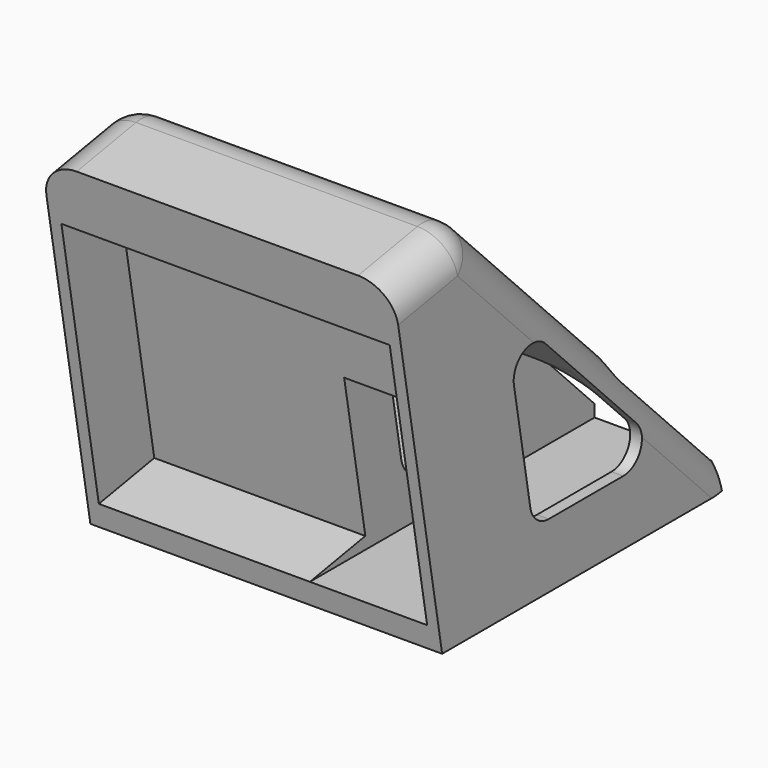
from build123d import *

# Parameters (mm, degrees)
F0_W          = 30
F0_H          = 30
F4_DEPTH      = 3
F3_W          = 30
F3_H          = 30
F5_DEPTH      = 8
F6_DEPTH      = 25
F8_DEPTH      = 6.0000000522
F10_DEPTH     = 30
F7_W          = 10
F7_H          = 11.7721162952
F7_H_2        = 1.030384494
F11_DEPTH     = 35.21044533
F12_T4_DEPTH  = 18.4976166065
F12_T10_DEPTH = 18.4976166065
F12_T15_DEPTH = 17.5385665297
F12_T20_DEPTH = 17.5385665297
F12_T26_DEPTH = 17.5385665297
F12_T31_DEPTH = 17.5385665297
F12_T37_DEPTH = 18.4976166065
F12_T43_DEPTH = 18.4976166065
F12_T45_DEPTH = 13.9174578279
F12_T47_DEPTH = 24
F12_T49_DEPTH = 44.997612514
F12_T54_DEPTH = 3
F12_T60_DEPTH = 3
F3_W_2        = 10
F3_H_2        = 13
F13_DEPTH     = 5.1313021672
F14_DEPTH     = 10.5


# Not quite as in the source:
# - a fillet or chamfer that OpenCascade refuses, or shapes differently, is made with other operations: its cross-section is extruded or revolved along the edge and cut away or added


with BuildPart() as f4:
    # F0 (on Top) → F4 (new body)
    with BuildSketch(Plane.XY):
        with Locations((0, 15)):
            Rectangle(F0_W, F0_H)
    extrude(amount=F4_DEPTH)

    # F3 (on 3pt) → F5 (join)
    with BuildSketch(Plane(origin=(0, 0, 0), x_dir=(-1, 0, 0), z_dir=(0, 0.984807753, 0.1736481777))):
        with Locations((0, 15)):
            Rectangle(F3_W, F3_H)
        Polygon((-14, 2), (-14, 15), (-14, 25), (14, 25), (14, 2), (-4, 2), align=None, mode=Mode.SUBTRACT)
        Polygon((-14, 25), (-14, 15), (-4, 15), (-4, 2), (14, 2), (14, 25), align=None)
    extrude(amount=F5_DEPTH)

    # F0 (on Top) → F6 (cut)
    with BuildSketch(Plane.XY):
        with Locations((0, 15)):
            Rectangle(F0_W, F0_H)
    extrude(amount=-F6_DEPTH, mode=Mode.SUBTRACT)

    # F3 (on 3pt) → F8 (cut)
    with BuildSketch(Plane(origin=(0, 0, 0), x_dir=(-1, 0, 0), z_dir=(0, 0.984807753, 0.1736481777))):
        Polygon((-14, 25), (-14, 15), (-4, 15), (-4, 2), (14, 2), (14, 25), align=None)
    extrude(amount=F8_DEPTH, mode=Mode.SUBTRACT)

    # F9 (on face) → F10 (join, through all)
    with BuildSketch(Plane.YZ.offset(15)):
        Polygon((30, 3), (2.6690166941, 30.9334180117), (7.594431953, 3), align=None)
        with BuildLine():
            ThreePointArc((11.3703802933, 5.5), (10.0848050739, 5.9679111138), (9.4007647872, 7.1527036447))
            Line((9.4007647872, 7.1527036447), (7.6573020205, 17.0403723366))
            ThreePointArc((7.6573020205, 17.0403723366), (8.7131028501, 19.1666972856), (11.0564624317, 18.7863828744))
            Line((11.0564624317, 18.7863828744), (20.7308856563, 8.8987141825))
            ThreePointArc((20.7308856563, 8.8987141825), (21.1449009434, 6.7245737833), (19.3013407511, 5.5))
            Line((19.3013407511, 5.5), (11.3703802933, 5.5))
        make_face(mode=Mode.SUBTRACT)
    extrude(amount=-F10_DEPTH)

    # F7 (on face) → F11 (cut, through all)
    with BuildSketch(Plane(origin=(0, 30, 0), x_dir=(-1, 0, 0), z_dir=(0, 1, 0))):
        with Locations((-9, 8.8860581476)):
            Rectangle(F7_W, F7_H)
        with Locations((-9, 2.484807753)):
            Rectangle(F7_W, F7_H_2)
    extrude(amount=-F11_DEPTH, mode=Mode.SUBTRACT)

    # F12: fillet of radius 3 on 9 edges, made by hand


with BuildPart() as f12_tool2:
    # F12_s3 → F12_t4 (new body)
    with BuildSketch(Plane.XZ.offset(-25.9817706947)):
        with BuildLine():
            ThreePointArc((7, 14.7721162952), (4.8786796564, 13.8934366387), (4, 11.7721162952))
            Line((4, 11.7721162952), (4, 14.7721162952))
            Line((4, 14.7721162952), (7, 14.7721162952))
        make_face()
    extrude(amount=F12_T4_DEPTH)

    split(bisect_by=Plane(origin=(0, 16.8266333185, 16.4637365227), x_dir=(1, 0, 0), z_dir=(0, -0.7147724526, -0.6993570912)), keep=Keep.TOP)

    split(bisect_by=Plane(origin=(0, 15.0397021871, 14.7153437946), x_dir=(1, 0, 0), z_dir=(0, 0.7147724526, 0.6993570912)), keep=Keep.TOP)


with BuildPart() as f4_1:
    add(f4.part)

    # F12_t1: union F12_tool2
    add(f12_tool2.part)


with BuildPart() as f12_tool8:
    # F12_s9 → F12_t10 (new body)
    with BuildSketch(Plane.XZ.offset(-25.9817706947)):
        with BuildLine():
            ThreePointArc((7, 14.7721162952), (4.8786796564, 13.8934366387), (4, 11.7721162952))
            Line((4, 11.7721162952), (4, 14.7721162952))
            Line((4, 14.7721162952), (7, 14.7721162952))
        make_face()
    extrude(amount=F12_T10_DEPTH)

    split(bisect_by=Plane(origin=(0, 10.3404814066, 1.8233058655), x_dir=(1, 0, 0), z_dir=(0, -0.984807753, -0.1736481777)), keep=Keep.TOP)


with BuildPart() as f4_2:
    add(f4_1.part)

    # F12_t7: union F12_tool8
    add(f12_tool8.part)


with BuildPart() as f12_tool13:
    # F12_s14 → F12_t15 (new body)
    with BuildSketch(Plane.XZ.offset(-15.5572567598)):
        with BuildLine():
            ThreePointArc((7, 14.7721162952), (4.8786796564, 13.8934366387), (4, 11.7721162952))
            Line((4, 11.7721162952), (4, 14.7721162952))
            Line((4, 14.7721162952), (7, 14.7721162952))
        make_face()
    extrude(amount=F12_T15_DEPTH)

    split(bisect_by=Plane(origin=(0, 15.0397021871, 14.7153437946), x_dir=(1, 0, 0), z_dir=(0, 0.7147724526, 0.6993570912)), keep=Keep.TOP)


with BuildPart() as f4_3:
    add(f4_2.part)

    # F12_t12: union F12_tool13
    add(f12_tool13.part)


with BuildPart() as f12_tool18:
    # F12_s19 → F12_t20 (new body)
    with BuildSketch(Plane.XZ.offset(-15.5572567598)):
        with BuildLine():
            ThreePointArc((7, 14.7721162952), (4.8786796564, 13.8934366387), (4, 11.7721162952))
            Line((4, 11.7721162952), (4, 14.7721162952))
            Line((4, 14.7721162952), (7, 14.7721162952))
        make_face()
    extrude(amount=F12_T20_DEPTH)

    split(bisect_by=Plane(origin=(0, 10.3404814066, 1.8233058655), x_dir=(1, 0, 0), z_dir=(0, -0.984807753, -0.1736481777)), keep=Keep.TOP)

    split(bisect_by=Plane(origin=(0, 7.8784620241, 1.3891854213), x_dir=(1, 0, 0), z_dir=(0, 0.984807753, 0.1736481777)), keep=Keep.TOP)


with BuildPart() as f4_4:
    add(f4_3.part)

    # F12_t17: union F12_tool18
    add(f12_tool18.part)


with BuildPart() as f12_tool24:
    # F12_s25 → F12_t26 (new body)
    with BuildSketch(Plane.XZ.offset(-15.5572567598)):
        with BuildLine():
            ThreePointArc((14, 11.7721162952), (13.1213203436, 13.8934366387), (11, 14.7721162952))
            Line((11, 14.7721162952), (14, 14.7721162952))
            Line((14, 14.7721162952), (14, 11.7721162952))
        make_face()
    extrude(amount=F12_T26_DEPTH)

    split(bisect_by=Plane(origin=(0, 15.0397021871, 14.7153437946), x_dir=(1, 0, 0), z_dir=(0, 0.7147724526, 0.6993570912)), keep=Keep.TOP)


with BuildPart() as f4_5:
    add(f4_4.part)

    # F12_t23: union F12_tool24
    add(f12_tool24.part)


with BuildPart() as f12_tool29:
    # F12_s30 → F12_t31 (new body)
    with BuildSketch(Plane.XZ.offset(-15.5572567598)):
        with BuildLine():
            ThreePointArc((14, 11.7721162952), (13.1213203436, 13.8934366387), (11, 14.7721162952))
            Line((11, 14.7721162952), (14, 14.7721162952))
            Line((14, 14.7721162952), (14, 11.7721162952))
        make_face()
    extrude(amount=F12_T31_DEPTH)

    split(bisect_by=Plane(origin=(0, 10.3404814066, 1.8233058655), x_dir=(1, 0, 0), z_dir=(0, -0.984807753, -0.1736481777)), keep=Keep.TOP)

    split(bisect_by=Plane(origin=(0, 7.8784620241, 1.3891854213), x_dir=(1, 0, 0), z_dir=(0, 0.984807753, 0.1736481777)), keep=Keep.TOP)


with BuildPart() as f4_6:
    add(f4_5.part)

    # F12_t28: union F12_tool29
    add(f12_tool29.part)


with BuildPart() as f12_tool35:
    # F12_s36 → F12_t37 (new body)
    with BuildSketch(Plane.XZ.offset(-25.9817706947)):
        with BuildLine():
            ThreePointArc((14, 11.7721162952), (13.1213203436, 13.8934366387), (11, 14.7721162952))
            Line((11, 14.7721162952), (14, 14.7721162952))
            Line((14, 14.7721162952), (14, 11.7721162952))
        make_face()
    extrude(amount=F12_T37_DEPTH)

    split(bisect_by=Plane(origin=(0, 16.8266333185, 16.4637365227), x_dir=(1, 0, 0), z_dir=(0, -0.7147724526, -0.6993570912)), keep=Keep.TOP)

    split(bisect_by=Plane(origin=(0, 15.0397021871, 14.7153437946), x_dir=(1, 0, 0), z_dir=(0, 0.7147724526, 0.6993570912)), keep=Keep.TOP)


with BuildPart() as f4_7:
    add(f4_6.part)

    # F12_t34: union F12_tool35
    add(f12_tool35.part)


with BuildPart() as f12_tool41:
    # F12_s42 → F12_t43 (new body)
    with BuildSketch(Plane.XZ.offset(-25.9817706947)):
        with BuildLine():
            ThreePointArc((14, 11.7721162952), (13.1213203436, 13.8934366387), (11, 14.7721162952))
            Line((11, 14.7721162952), (14, 14.7721162952))
            Line((14, 14.7721162952), (14, 11.7721162952))
        make_face()
    extrude(amount=F12_T43_DEPTH)

    split(bisect_by=Plane(origin=(0, 10.3404814066, 1.8233058655), x_dir=(1, 0, 0), z_dir=(0, -0.984807753, -0.1736481777)), keep=Keep.TOP)


with BuildPart() as f4_8:
    add(f4_7.part)

    # F12_t40: union F12_tool41
    add(f12_tool41.part)

    # F12_s46 → F12_t45 (cut)
    with BuildSketch(Plane(origin=(0, -7.3860581476, -1.3023613325), x_dir=(1, 0, 0), z_dir=(0, 0.984807753, 0.1736481777))):
        with BuildLine():
            ThreePointArc((-15, -27), (-14.1213203436, -29.1213203436), (-12, -30))
            Line((-12, -30), (-15, -30))
            Line((-15, -30), (-15, -27))
        make_face()
        with BuildLine():
            ThreePointArc((15, -27), (14.1213203436, -29.1213203436), (12, -30))
            Line((12, -30), (15, -30))
            Line((15, -30), (15, -27))
        make_face()
    extrude(amount=F12_T45_DEPTH, mode=Mode.SUBTRACT)

    # F12_s48 → F12_t47 (cut)
    with BuildSketch(Plane.YZ.offset(-12)):
        with BuildLine():
            ThreePointArc((1.1105168936, 30.6586124474), (2.5491593686, 30.5603807939), (3.7757787843, 29.8022604621))
            Line((3.7757787843, 29.8022604621), (2.6690166941, 30.9334180117))
            Line((2.6690166941, 30.9334180117), (1.1105168936, 30.6586124474))
        make_face()
    extrude(amount=F12_T47_DEPTH, mode=Mode.SUBTRACT)

    # F12_s50 → F12_t49 (cut)
    with BuildSketch(Plane(origin=(0, 18.4185448657, -18.8245299169), x_dir=(1, 0, 0), z_dir=(0, -0.6993570912, 0.7147724526))):
        with BuildLine():
            ThreePointArc((-15, 20.5412448507), (-14.1213203436, 22.6625651943), (-12, 23.5412448507))
            Line((-12, 23.5412448507), (-15, 23.5412448507))
            Line((-15, 23.5412448507), (-15, 20.5412448507))
        make_face()
        with BuildLine():
            ThreePointArc((15, 20.5412448507), (14.1213203436, 22.6625651943), (12, 23.5412448507))
            Line((12, 23.5412448507), (15, 23.5412448507))
            Line((15, 23.5412448507), (15, 20.5412448507))
        make_face()
    extrude(amount=F12_T49_DEPTH, mode=Mode.SUBTRACT)


with BuildPart() as f12_tool52:
    # F12_s53 → F12_t54 (new body)
    with BuildSketch(Plane.YZ.offset(-12)):
        Polygon((1.6314614266, 27.7041891884), (1.1105168936, 30.6586124474), (2.6690166941, 30.9334180117), (3.7757787843, 29.8022604621), align=None)
    extrude(amount=-F12_T54_DEPTH)

    # F12_s55 → F12_t56 (revolve, cut)
    with BuildSketch(Plane(origin=(-12, 1.6314614266, 27.7041891884), x_dir=(0, -0.305899314, -0.9520638685), z_dir=(0, 0.9520638685, -0.305899314))):
        with BuildLine():
            ThreePointArc((0, -3), (3, 0), (0, 3))
            Line((0, 3), (0, -3))
        make_face()
    revolve(axis=Axis((-12, 1.6314614266, 27.7041891884), (-1, 0, 0)), mode=Mode.SUBTRACT)


with BuildPart() as f4_9:
    add(f4_8.part)

    # F12_t51: cut F12_tool52
    add(f12_tool52.part, mode=Mode.SUBTRACT)


with BuildPart() as f12_tool58:
    # F12_s59 → F12_t60 (new body)
    with BuildSketch(Plane.YZ.offset(12)):
        Polygon((1.6314614266, 27.7041891884), (3.7757787843, 29.8022604621), (2.6690166941, 30.9334180117), (1.1105168936, 30.6586124474), align=None)
    extrude(amount=F12_T60_DEPTH)

    # F12_s61 → F12_t62 (revolve, cut)
    with BuildSketch(Plane(origin=(12, 1.6314614266, 27.7041891884), x_dir=(0, -0.305899314, -0.9520638685), z_dir=(0, -0.9520638685, 0.305899314))):
        with BuildLine():
            ThreePointArc((0, -3), (3, 0), (0, 3))
            Line((0, 3), (0, -3))
        make_face()
    revolve(axis=Axis((12, 1.6314614266, 27.7041891884), (1, 0, 0)), mode=Mode.SUBTRACT)


with BuildPart() as f4_10:
    add(f4_9.part)

    # F12_t57: cut F12_tool58
    add(f12_tool58.part, mode=Mode.SUBTRACT)

    # F3 (on 3pt) → F13 (cut, through all)
    with BuildSketch(Plane(origin=(0, 0, 0), x_dir=(-1, 0, 0), z_dir=(0, 0.984807753, 0.1736481777))):
        with Locations((0, 15)):
            Rectangle(F3_W, F3_H)
        Polygon((-14, 2), (-14, 15), (-14, 25), (14, 25), (14, 2), (-4, 2), align=None, mode=Mode.SUBTRACT)
        Polygon((-14, 25), (-14, 15), (-4, 15), (-4, 2), (14, 2), (14, 25), align=None)
        with Locations((-9, 8.5)):
            Rectangle(F3_W_2, F3_H_2)
    extrude(amount=-F13_DEPTH, mode=Mode.SUBTRACT)

    # F3 (on 3pt) → F14 (cut, through all)
    with BuildSketch(Plane(origin=(0, 0, 0), x_dir=(-1, 0, 0), z_dir=(0, 0.984807753, 0.1736481777))):
        with Locations((-9, 8.5)):
            Rectangle(F3_W_2, F3_H_2)
    extrude(amount=F14_DEPTH, mode=Mode.SUBTRACT)


solid = f4_10.part
